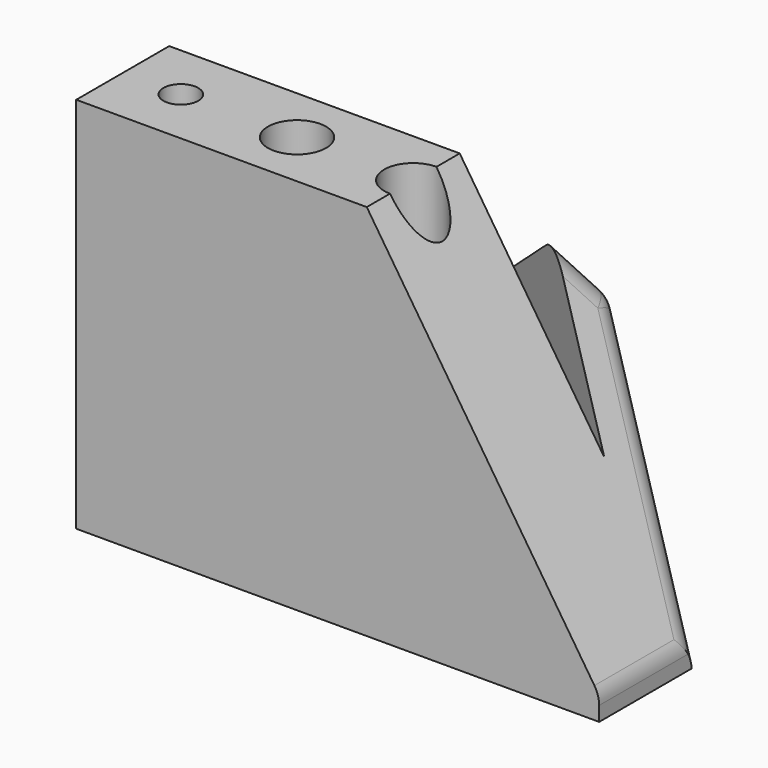
from build123d import *

# Parameters (mm, degrees)
F1_DEPTH      = 65
F3_DEPTH      = 60.001
F5_DEPTH      = 90.001
F6_R          = 2.5
F6_R_2        = 2.6062767238
F6_R_3        = 2.7274571226
F6_R_4        = 2.3400008441
F6_R_5        = 2.2698965194
F7_DEPTH      = 65.001
F8_R          = 5
F9_DEPTH      = 61
F10_T1_DEPTH  = 54.6888355079
F10_T3_DEPTH  = 66.0983799095
F10_T5_DEPTH  = 27.4657405621
F10_T7_DEPTH  = 27.4657405621
F10_T9_DEPTH  = 19.6621717152
F10_T14_DEPTH = 7.5244057305
F11_R         = 3
F12_DEPTH     = 65.001


# Not quite as in the source:
# - a fillet or chamfer that OpenCascade refuses, or shapes differently, is made with other operations: its cross-section is extruded or revolved along the edge and cut away or added


with BuildPart() as f1:
    # F0 (on Top) → F1 (new body)
    with BuildSketch(Plane.XY):
        Polygon((0, 60), (0, 0), (90, 0), (90, 20), (20, 60), align=None)
        Polygon((74.8832667219, 20), (20, 20), (20, 51.3618666983), align=None, mode=Mode.SUBTRACT)
    extrude(amount=F1_DEPTH)

    # F2 (on face) → F3 (cut, through all)
    with BuildSketch(Plane.XZ):
        Polygon((90, 65), (50, 65), (90, 4), align=None)
    extrude(amount=-F3_DEPTH, mode=Mode.SUBTRACT)

    # F4 (on face) → F5 (cut, through all)
    with BuildSketch(Plane(origin=(0, 0, 0), x_dir=(0, -1, 0), z_dir=(-1, 0, 0))):
        Polygon((-60, 65), (-60, 4), (-20, 65), align=None)
    extrude(amount=-F5_DEPTH, mode=Mode.SUBTRACT)

    # F6 (on face) → F7 (cut, through all)
    with BuildSketch(Plane(origin=(0, 0, 0), x_dir=(1, 0, 0), z_dir=(0, 0, -1))):
        with Locations((10, -10)):
            Circle(F6_R)
        with Locations((30, -10)):
            Circle(F6_R_2)
        with Locations((50, -10)):
            Circle(F6_R_3)
        with Locations((10, -30)):
            Circle(F6_R_4)
        with Locations((10, -50)):
            Circle(F6_R_5)
    extrude(amount=-F7_DEPTH, mode=Mode.SUBTRACT)

    # F8 (on face) → F9 (cut)
    with BuildSketch(Plane.XY.offset(65)):
        with Locations((30, 10)):
            Circle(F8_R)
        with Locations((50, 10)):
            Circle(F8_R)
        with Locations((10, 30)):
            Circle(F8_R)
        with Locations((10, 50)):
            Circle(F8_R)
    extrude(amount=-F9_DEPTH, mode=Mode.SUBTRACT)

    # F10: fillet of radius 5 on 5 edges, made by hand

    # F10_s2 → F10_t1 (cut)
    with BuildSketch(Plane(origin=(-4.5673183312, 2.6098961893, 6.9651604551), x_dir=(0.4961389384, 0.8682431421, 0), z_dir=(0.5232694295, -0.2990111026, -0.79798588))):
        with BuildLine():
            ThreePointArc((62.0173672946, 53.6332556425), (61.2228598232, 56.3376654842), (59.0918342578, 58.1826057959))
            Line((59.0918342578, 58.1826057959), (62.0173672946, 56.848586336))
            Line((62.0173672946, 56.848586336), (62.0173672946, 53.6332556425))
        make_face()
    extrude(amount=F10_T1_DEPTH, mode=Mode.SUBTRACT)

    # F10_s4 → F10_t3 (cut)
    with BuildSketch(Plane(origin=(-8.625501954, 4.9288582594, -7.5165088456), x_dir=(0.4961389384, 0.8682431421, 0), z_dir=(0.6923908912, -0.3956519378, 0.6033692052))):
        with BuildLine():
            ThreePointArc((60.6476844802, 12.1199645789), (61.6623423176, 10.5322872681), (62.0173672946, 8.6818259645))
            Line((62.0173672946, 8.6818259645), (62.0173672946, 10.6737218244))
            Line((62.0173672946, 10.6737218244), (60.6476844802, 12.1199645789))
        make_face()
    extrude(amount=F10_T3_DEPTH, mode=Mode.SUBTRACT)

    # F10_s6 → F10_t5 (cut)
    with BuildSketch(Plane.XZ.offset(-23.732870281)):
        with BuildLine():
            ThreePointArc((90, 2.5068518876), (89.7909346262, 3.9375668863), (89.1812218369, 5.2486366987))
            Line((89.1812218369, 5.2486366987), (90, 4))
            Line((90, 4), (90, 2.5068518876))
        make_face()
    extrude(amount=F10_T5_DEPTH, mode=Mode.SUBTRACT)

    # F10_s8 → F10_t7 (cut)
    with BuildSketch(Plane.YZ.offset(-3.732870281)):
        with BuildLine():
            ThreePointArc((59.1812218369, 5.2486366987), (59.7909346262, 3.9375668863), (60, 2.5068518876))
            Line((60, 2.5068518876), (60, 4))
            Line((60, 4), (59.1812218369, 5.2486366987))
        make_face()
    extrude(amount=F10_T7_DEPTH, mode=Mode.SUBTRACT)

    # F10_s10 → F10_t9 (cut)
    with BuildSketch(Plane(origin=(7.3622659095, 7.3622659095, -11.227455512), x_dir=(0.7071067812, -0.7071067812, 0), z_dir=(-0.4808122973, -0.4808122973, 0.7332387534))):
        with BuildLine():
            ThreePointArc((18.2566331211, 78.32372737), (21.2132034356, 79.2915205331), (24.1697737501, 78.32372737))
            Line((24.1697737501, 78.32372737), (21.2132034356, 80.4915993018))
            Line((21.2132034356, 80.4915993018), (18.2566331211, 78.32372737))
        make_face()
    extrude(amount=F10_T9_DEPTH, mode=Mode.SUBTRACT)


with BuildPart() as f10_tool12:
    # F10_s13 → F10_t14 (new body)
    with BuildSketch(Plane(origin=(40.048894076, 51.2336348167, 32.9651231761), x_dir=(-0.7878556137, 0.6158599938, 0), z_dir=(0.5493112883, 0.7027213758, 0.4521501704))):
        Polygon((-33.23229157, 16.8297290824), (-38.6871469703, 2.8043492675), (-24.6617671554, -2.6505061327), (-19.2069117551, 11.3748736822), align=None)
    extrude(amount=F10_T14_DEPTH)

    split(bisect_by=Plane(origin=(7.3622659095, 7.3622659095, -11.227455512), x_dir=(-0.7071067812, 0.7071067812, 0), z_dir=(0.4808122973, 0.4808122973, -0.7332387534)), keep=Keep.TOP)

    split(bisect_by=Plane(origin=(37.1404142209, -21.2230938405, 32.3652181067), x_dir=(0.4961389384, 0.8682431421, 0), z_dir=(0.6923908912, -0.3956519378, 0.6033692052)), keep=Keep.TOP)

    split(bisect_by=Plane(origin=(-4.5673183312, 2.6098961893, 6.9651604551), x_dir=(-0.4961389384, -0.8682431421, 0), z_dir=(-0.5232694295, 0.2990111026, 0.79798588)), keep=Keep.TOP)

    split(bisect_by=Plane(origin=(64.7716594625, 0, 42.4732193197), x_dir=(0, 1, 0), z_dir=(-0.8362443674, 0, -0.5483569622)), keep=Keep.TOP)

    split(bisect_by=Plane(origin=(0, 43.792520203, 28.7164066905), x_dir=(1, 0, 0), z_dir=(0, -0.8362443674, -0.5483569622)), keep=Keep.TOP)

    split(bisect_by=Plane(origin=(30.7692307692, 53.8461538462, 0), x_dir=(0, 0, 1), z_dir=(-0.4961389384, -0.8682431421, 0)), keep=Keep.TOP)

    # F10_s21 → F10_t22 (revolve, cut)
    with BuildSketch(Plane(origin=(60.8807919326, 30.8807919326, 39.2886441904), x_dir=(-0.5493112883, -0.7027213758, -0.4521501704), z_dir=(0.6333396268, -0.7031019234, 0.3233088345))):
        with BuildLine():
            ThreePointArc((0, -5), (5, 0), (0, 5))
            Line((0, 5), (0, -5))
        make_face()
    revolve(axis=Axis((60.8807919326, 30.8807919326, 39.2886441904), (0.5451036834, 0.1087674278, -0.8312831172)), mode=Mode.SUBTRACT)


with BuildPart() as f1_1:
    add(f1.part)

    # F10_t11: cut F10_tool12
    add(f10_tool12.part, mode=Mode.SUBTRACT)

    # F11 (on face) → F12 (cut, through all)
    with BuildSketch(Plane(origin=(0, 0, 0), x_dir=(1, 0, 0), z_dir=(0, 0, -1))):
        with Locations((10, -10)):
            Circle(F11_R)
    extrude(amount=-F12_DEPTH, mode=Mode.SUBTRACT)


solid = f1_1.part
